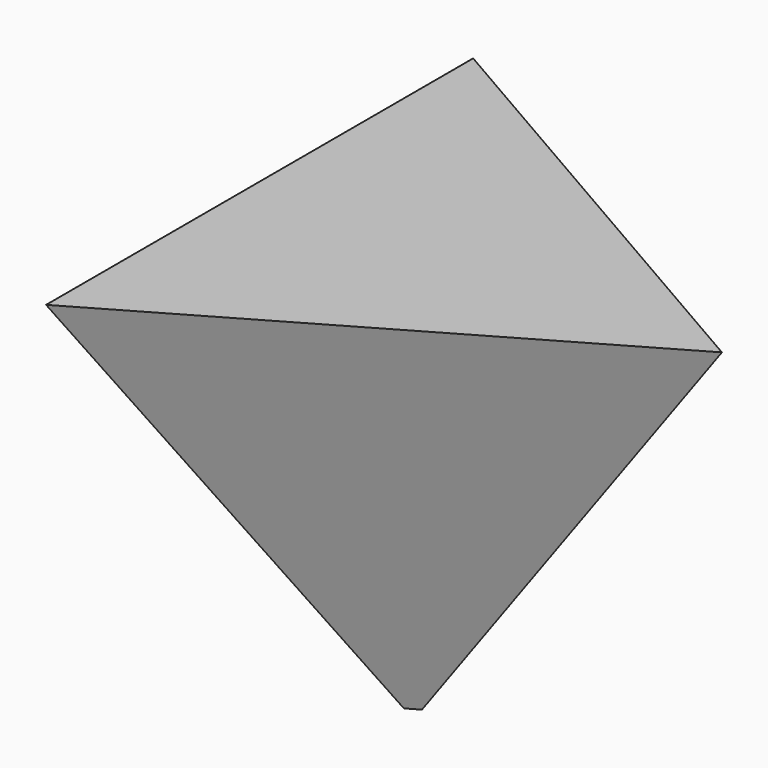
from build123d import *

# Parameters (mm, degrees)
F1_DEPTH = 1000
F1_TAPER = -20


with BuildPart() as f1:
    # F0 (on Top) → F1 (new body)
    with BuildSketch(Plane.XY):
        Polygon((20, 0), (-10, 17.3205080757), (-10, -17.3205080757), align=None)
    extrude(amount=F1_DEPTH, taper=F1_TAPER)


solid = f1.part
